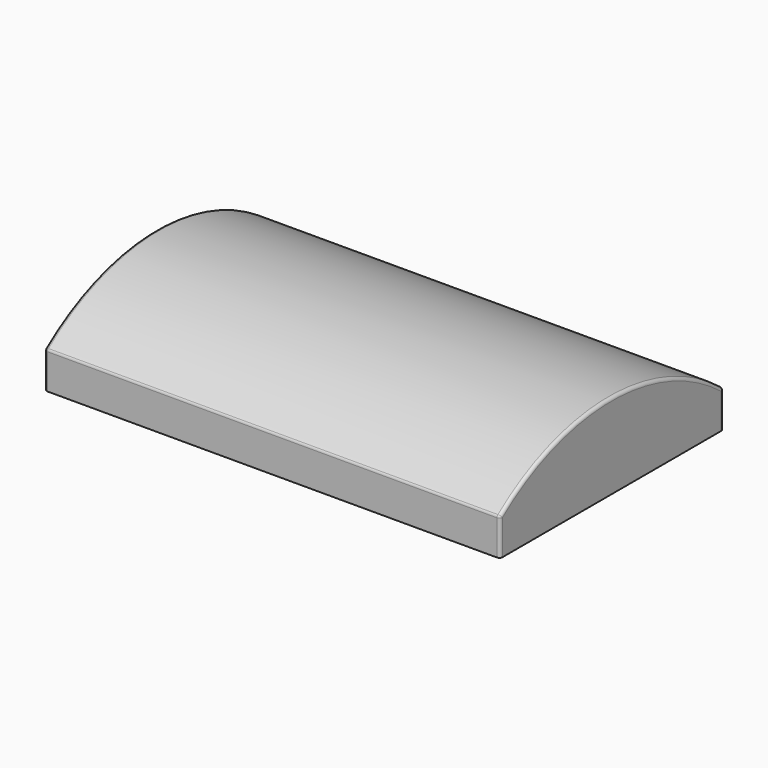
from build123d import *

# Parameters (mm, degrees)
F1_DEPTH = 750
F2_DEPTH = 10
F6_R     = 5


# Not quite as in the source:
# - a feature of the source that left no trace in its solid (it failed there, or was rolled back) is left out


with BuildPart() as f1:
    # F0 (on Right) → F1 (new body)
    with BuildSketch(Plane.YZ):
        with BuildLine():
            Line((-213.512294728, 30), (-230, 30))
            Line((-230, 30), (-230, -30))
            Line((-230, -30), (-220, -30))
            Line((-220, -30), (-220, 25.1203247649))
            ThreePointArc((-220, 25.1203247649), (-216.7698785064, 27.5784184345), (-213.512294728, 30))
        make_face()
        with BuildLine():
            ThreePointArc((230, 30), (0, 110), (-230, 30))
            Line((-230, 30), (-213.512294728, 30))
            ThreePointArc((-213.512294728, 30), (0, 100), (213.512294728, 30))
            Line((213.512294728, 30), (230, 30))
        make_face()
        with BuildLine():
            Line((230, -30), (230, 30))
            Line((230, 30), (213.512294728, 30))
            ThreePointArc((213.512294728, 30), (216.7698785064, 27.5784184345), (220, 25.1203247649))
            Line((220, 25.1203247649), (220, -30))
            Line((220, -30), (230, -30))
        make_face()
    extrude(amount=F1_DEPTH)

    # F0 (on Right) → F2 (join)
    with BuildSketch(Plane.YZ):
        with BuildLine():
            ThreePointArc((230, 30), (0, 110), (-230, 30))
            Line((-230, 30), (-213.512294728, 30))
            ThreePointArc((-213.512294728, 30), (0, 100), (213.512294728, 30))
            Line((213.512294728, 30), (230, 30))
        make_face()
        with BuildLine():
            Line((-213.512294728, 30), (-230, 30))
            Line((-230, 30), (-230, -30))
            Line((-230, -30), (-220, -30))
            Line((-220, -30), (-220, 25.1203247649))
            ThreePointArc((-220, 25.1203247649), (-216.7698785064, 27.5784184345), (-213.512294728, 30))
        make_face()
        with BuildLine():
            Line((213.512294728, 30), (-213.512294728, 30))
            ThreePointArc((-213.512294728, 30), (-216.7698785064, 27.5784184345), (-220, 25.1203247649))
            Line((-220, 25.1203247649), (-220, -30))
            Line((-220, -30), (220, -30))
            Line((220, -30), (220, 25.1203247649))
            ThreePointArc((220, 25.1203247649), (216.7698785064, 27.5784184345), (213.512294728, 30))
        make_face()
        with BuildLine():
            ThreePointArc((213.512294728, 30), (0, 100), (-213.512294728, 30))
            Line((-213.512294728, 30), (213.512294728, 30))
        make_face()
        with BuildLine():
            Line((230, -30), (230, 30))
            Line((230, 30), (213.512294728, 30))
            ThreePointArc((213.512294728, 30), (216.7698785064, 27.5784184345), (220, 25.1203247649))
            Line((220, 25.1203247649), (220, -30))
            Line((220, -30), (230, -30))
        make_face()
    extrude(amount=F2_DEPTH)

    # F4: F1 across plane


with BuildPart() as f1_1:
    add(f1.part)
    add(f1.part.mirror(Plane.YZ.offset(375)))

    # F6
    f6_edges = [f1_1.edges().sort_by_distance(p)[0] for p in [
        (750, 0, 110),
        (375, 230, 30),
        (0, 0, 110),
        (375, -230, 30),
        (0, -230, 0),
        (750, -230, 0),
        (0, 230, 0),
        (750, 230, 0),
    ]]
    fillet(f6_edges, radius=F6_R)


solid = f1_1.part
